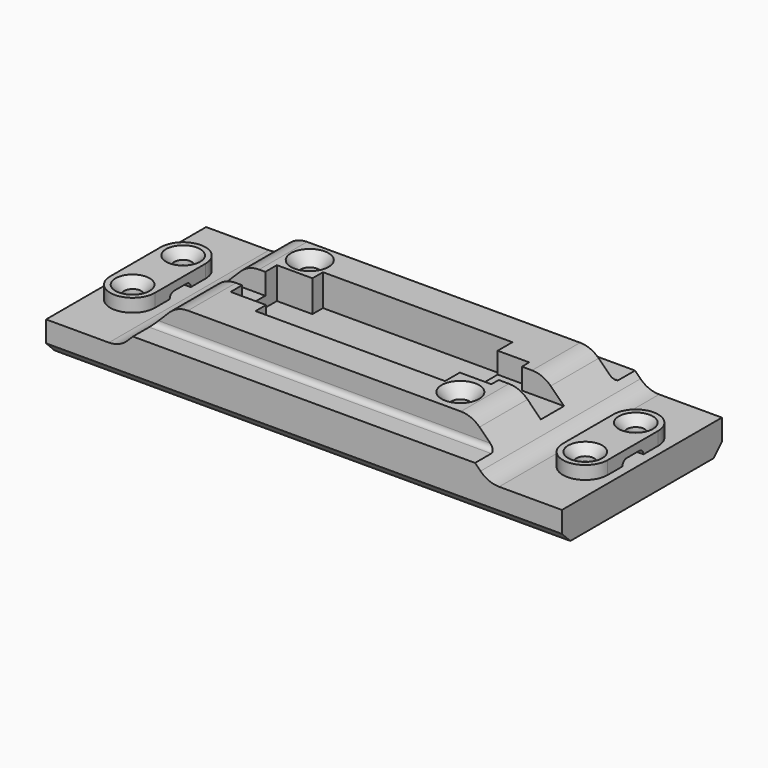
from build123d import *

# Parameters (mm, degrees)
F1_DEPTH               = 70
F2_SIZE                = 2
F3_R                   = 1
F5_SIZE                = 7
F6_DEPTH               = 14
F7_DEPTH               = 14
F8_R                   = 5
F4_W                   = 36
F4_H                   = 16
F9_DEPTH               = 6
F10_W                  = 11
F10_H                  = 6
F11_DEPTH              = 6.75
F12_W                  = 9
F12_H                  = 4
F13_DEPTH              = 6
F14_W                  = 5.5
F14_H                  = 4
F15_DEPTH              = 8.001
F17_W                  = 5.5
F17_H                  = 4
F18_DEPTH              = 7.251
F20_D                  = 3
F20_DEPTH              = 13.8
F20_TIP                = 0.9012909285
F20_ON_F19_D           = 3
F20_ON_F19_DEPTH       = 13.8
F20_ON_F19_TIP         = 0.9012909285
F23_D                  = 3.4544
F23_DEPTH              = 14.4
F23_CSINK_D            = 7.1374
F23_CSINK_ANGLE        = 82
F23_TIP                = 1.0378064612
F23_ON_F22_D           = 3.4544
F23_ON_F22_DEPTH       = 14.4
F23_ON_F22_CSINK_D     = 7.1374
F23_ON_F22_CSINK_ANGLE = 82
F23_ON_F22_TIP         = 1.0378064612
F25_DEPTH              = 2.5
F27_W                  = 8.5
F27_H                  = 5
F28_DEPTH              = 1
F29_R                  = 0.99999
F30_D                  = 3.3
F30_DEPTH              = 14.4
F30_CSINK_D            = 6.5
F30_CSINK_ANGLE        = 90
F30_TIP                = 0.9914200214


# Not quite as in the source:
# - a fillet or chamfer is up to 0.001 mm smaller than in the source, because OpenCascade refuses the exact size


with BuildPart() as f1:
    # F0 (on Right) → F1 (new body)
    with BuildSketch(Plane.YZ):
        Polygon((-19, -4.25), (19, -4.25), (19, 4.25), (14.15, 4.25), (14.15, 8.75), (-14.15, 8.75), (-14.15, 4.25), (-19, 4.25), align=None)
    extrude(amount=F1_DEPTH)

    # F2
    f2_edges = [f1.edges().sort_by_distance(p)[0] for p in [
        (35, -19, -4.25),
        (35, 19, -4.25),
    ]]
    chamfer(f2_edges, length=F2_SIZE)

    # F3
    f3_edges = [f1.edges().sort_by_distance(p)[0] for p in [
        (35, 14.15, 4.25),
        (35, -14.15, 4.25),
    ]]
    fillet(f3_edges, radius=F3_R)

    # F5
    f5_edges = [f1.edges().sort_by_distance(p)[0] for p in [
        (70, 0, 8.75),
        (0, 0, 8.75),
    ]]
    chamfer(f5_edges, length=F5_SIZE)

    # F6 (add): a face of the model
    f6_faces = [f1.faces().sort_by_distance(p)[0] for p in [
        (0, 0, -1.2083333333),
    ]]
    extrude(f6_faces, amount=F6_DEPTH)

    # F7 (add): a face of the model
    f7_faces = [f1.faces().sort_by_distance(p)[0] for p in [
        (70, 0, -1.2083333333),
    ]]
    extrude(f7_faces, amount=F7_DEPTH)

    # F8
    f8_edges = [f1.edges().sort_by_distance(p)[0] for p in [
        (63, 0, 8.75),
        (70, 0, 1.75),
        (7, 0, 8.75),
        (0, 0, 1.75),
    ]]
    fillet(f8_edges, radius=F8_R)

    # F4 (on face) → F9 (cut)
    with BuildSketch(Plane.XY.offset(8.75)):
        with Locations((35, 0)):
            Rectangle(F4_W, F4_H)
    extrude(amount=-F9_DEPTH, mode=Mode.SUBTRACT)

    # F10 (on face) → F11 (cut)
    with BuildSketch(Plane.YZ.offset(17)):
        with Locations((0, 5.75)):
            Rectangle(F10_W, F10_H)
    extrude(amount=-F11_DEPTH, mode=Mode.SUBTRACT)

    # F12 (on face) → F13 (cut)
    with BuildSketch(Plane(origin=(53, 0, 0), x_dir=(0, -1, 0), z_dir=(-1, 0, 0))):
        with Locations((0, 6.75)):
            Rectangle(F12_W, F12_H)
    extrude(amount=-F13_DEPTH, mode=Mode.SUBTRACT)

    # F14 (on face) → F15 (cut, through all)
    with BuildSketch(Plane(origin=(59, 0, 0), x_dir=(0, -1, 0), z_dir=(-1, 0, 0))):
        with Locations((0, 6.75)):
            Rectangle(F14_W, F14_H)
    extrude(amount=-F15_DEPTH, mode=Mode.SUBTRACT)

    # F17 (on face) → F18 (cut, through all)
    with BuildSketch(Plane.YZ.offset(10.25)):
        with Locations((0, 6.75)):
            Rectangle(F17_W, F17_H)
    extrude(amount=-F18_DEPTH, mode=Mode.SUBTRACT)

    # F20
    with Locations(Plane.XY.offset(1.75)):
        with Locations((78.0355339059, -6), (78.0355339059, 6)):
            Hole(F20_D / 2, depth=F20_DEPTH)
            with Locations((0, 0, -(F20_DEPTH + F20_TIP / 2))):  # 118° drill point
                Cone(0, F20_D / 2, F20_TIP, mode=Mode.SUBTRACT)

    # F20 on F19
    with Locations(Plane.XY.offset(1.75)):
        with Locations((-8.0355339059, 6), (-8.0355339059, -6)):
            Hole(F20_ON_F19_D / 2, depth=F20_ON_F19_DEPTH)
            with Locations((0, 0, -(F20_ON_F19_DEPTH + F20_ON_F19_TIP / 2))):  # 118° drill point
                Cone(0, F20_ON_F19_D / 2, F20_ON_F19_TIP, mode=Mode.SUBTRACT)

    # F23
    with Locations(Plane.XY.offset(8.75)):
        with Locations((56.9644660941, -9.325)):
            CounterSinkHole(F23_D / 2, F23_CSINK_D / 2, depth=F23_DEPTH, counter_sink_angle=F23_CSINK_ANGLE)
            with Locations((0, 0, -(F23_DEPTH + F23_TIP / 2))):  # 118° drill point
                Cone(0, F23_D / 2, F23_TIP, mode=Mode.SUBTRACT)

    # F23 on F22
    with Locations(Plane.XY.offset(8.75)):
        with Locations((13.0355339059, 9.825)):
            CounterSinkHole(F23_ON_F22_D / 2, F23_ON_F22_CSINK_D / 2, depth=F23_ON_F22_DEPTH, counter_sink_angle=F23_ON_F22_CSINK_ANGLE)
            with Locations((0, 0, -(F23_ON_F22_DEPTH + F23_ON_F22_TIP / 2))):  # 118° drill point
                Cone(0, F23_ON_F22_D / 2, F23_ON_F22_TIP, mode=Mode.SUBTRACT)


with BuildPart() as f25:
    # F24 (on face) → F25 (new body)
    with BuildSketch(Plane.XY.offset(1.75)):
        with BuildLine():
            Line((73.7855339059, 6), (73.7855339059, -6))
            ThreePointArc((73.7855339059, -6), (78.0355339059, -10.25), (82.2855339059, -6))
            Line((82.2855339059, -6), (82.2855339059, 6))
            ThreePointArc((82.2855339059, 6), (78.0355339059, 10.25), (73.7855339059, 6))
        make_face()
    extrude(amount=F25_DEPTH)

    # F27 (on face) → F28 (cut)
    with BuildSketch(Plane.XY.offset(1.75)):
        with Locations((78.0355339059, 0)):
            Rectangle(F27_W, F27_H)
    extrude(amount=F28_DEPTH, mode=Mode.SUBTRACT)

    # F29 (radius 1 in the source; OpenCascade refuses exactly that, so slightly less here)
    f29_edges = [f25.edges().sort_by_distance(p)[0] for p in [
        (78.035534, 2.5, 2.75),
        (78.035534, -2.5, 2.75),
    ]]
    fillet(f29_edges, radius=F29_R)

    # F30
    with Locations(Plane.XY.offset(4.25)):
        with Locations((78.0355339059, -6), (78.0355339059, 6)):
            CounterSinkHole(F30_D / 2, F30_CSINK_D / 2, depth=F30_DEPTH, counter_sink_angle=F30_CSINK_ANGLE)
            with Locations((0, 0, -(F30_DEPTH + F30_TIP / 2))):  # 118° drill point
                Cone(0, F30_D / 2, F30_TIP, mode=Mode.SUBTRACT)


with BuildPart() as f31_1:
    # F31: copy of F25
    add(f25.part.moved(Location((-86, 0, 0))))


solid = Compound([f1.part, f25.part, f31_1.part])
